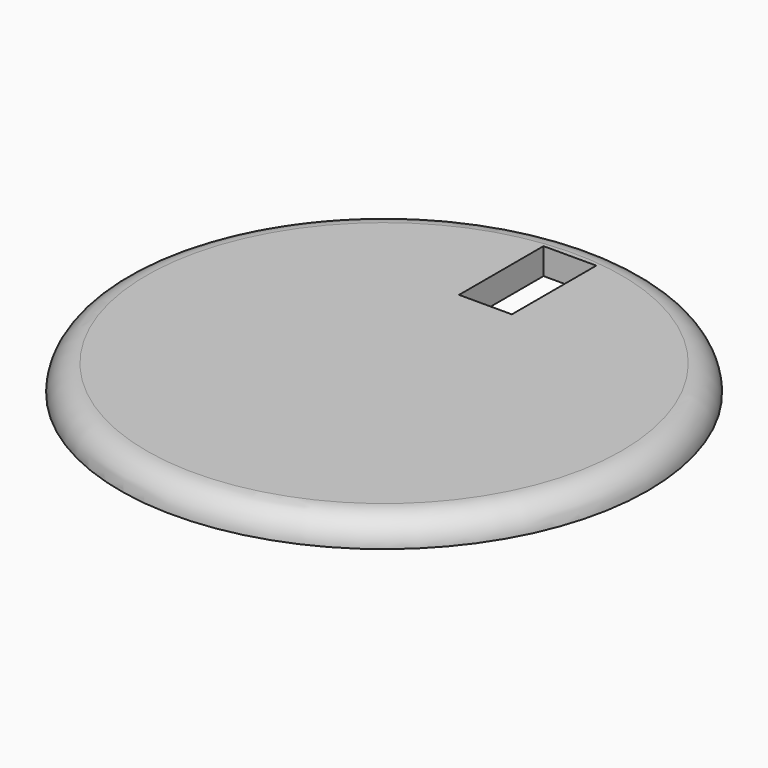
from build123d import *

# Parameters (mm, degrees)
F0_R     = 50
F0_W     = 10
F0_H     = 20
F1_DEPTH = 5
F2_R     = 4.99999


# Not quite as in the source:
# - a fillet or chamfer is up to 0.001 mm smaller than in the source, because OpenCascade refuses the exact size


with BuildPart() as f1:
    # F0 (on Top) → F1 (new body)
    with BuildSketch(Plane.XY):
        Circle(F0_R)
        with Locations((0, 34)):
            Rectangle(F0_W, F0_H, mode=Mode.SUBTRACT)
    extrude(amount=F1_DEPTH)

    # F2 (radius 5 in the source; OpenCascade refuses exactly that, so slightly less here)
    f2_edges = [f1.edges().sort_by_distance(p)[0] for p in [
        (-50, 0, 5),
    ]]
    fillet(f2_edges, radius=F2_R)


solid = f1.part
